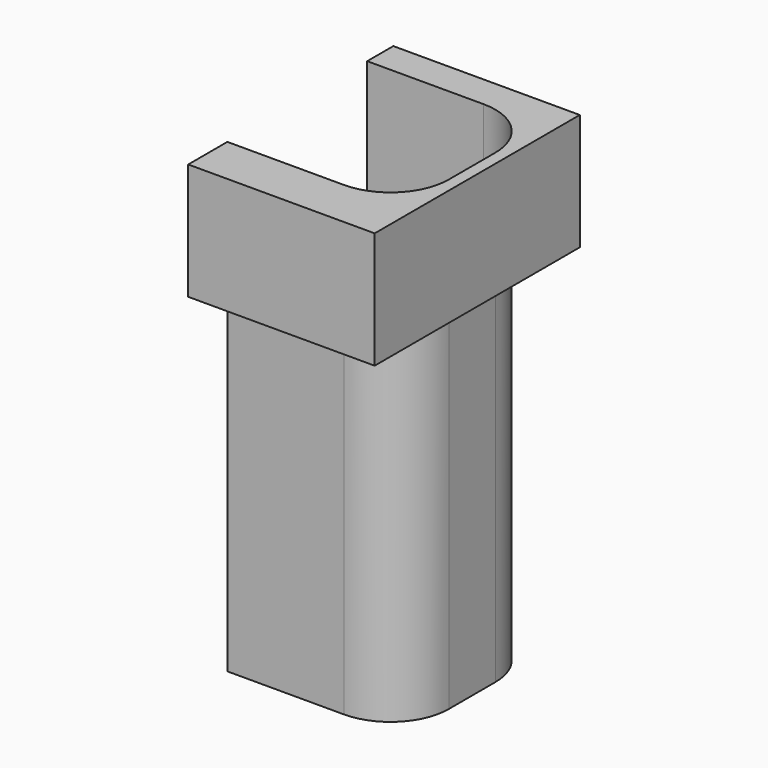
from build123d import *

# Parameters (mm, degrees)
F0_W     = 15
F0_H     = 15
F1_DEPTH = 30
F2_R     = 5
F4_DEPTH = 10


# Not quite as in the source:
# - ends of sketch curves that miss each other by under 0.0002 mm in the source are joined


with BuildPart() as f1:
    # F0 (on Top) → F1 (new body)
    with BuildSketch(Plane.XY):
        with Locations((7.5, 7.5)):
            Rectangle(F0_W, F0_H)
    extrude(amount=F1_DEPTH)

    # F2
    f2_edges = [f1.edges().sort_by_distance(p)[0] for p in [
        (15, 0, 15),
        (15, 15, 15),
    ]]
    fillet(f2_edges, radius=F2_R)


with BuildPart() as f4:
    # F3 (on face) → F4 (new body)
    with BuildSketch(Plane.XY.offset(30)):
        with BuildLine():
            Line((15.9999990687, -4.1973348707), (15.9999990687, 17.8026651293))
            Line((15.9999990687, 17.8026651293), (-9.313e-07, 17.8026651293))
            Line((-9.313e-07, 17.8026651293), (-9.313e-07, 15))
            Line((-9.313e-07, 15), (10, 15))
            ThreePointArc((10, 15), (13.5355339059, 13.5355339059), (15, 10))
            Line((15, 10), (15, 5))
            ThreePointArc((15, 5), (13.5355339059, 1.4644660941), (10, 0))
            Line((10, 0), (0, 0))
            Line((0, 0), (-9.313e-07, -4.1973348707))
            Line((-9.313e-07, -4.1973348707), (15.9999990687, -4.1973348707))
        make_face()
    extrude(amount=F4_DEPTH)


solid = Compound([f1.part, f4.part])
